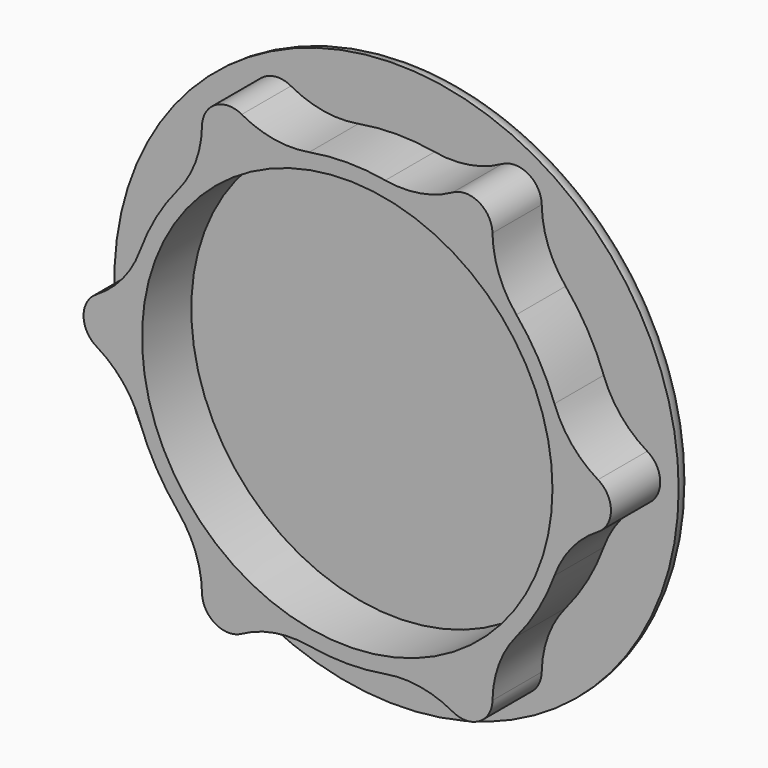
from build123d import *

# Parameters (mm, degrees)
F0_R     = 10
F1_DEPTH = 3
F2_R     = 13.75
F3_DEPTH = 1
F4_R     = 0.99999


# Not quite as in the source:
# - a fillet or chamfer is up to 0.001 mm smaller than in the source, because OpenCascade refuses the exact size


with BuildPart() as f1:
    # F0 (on Front) → F1 (new body)
    with BuildSketch(Plane.XZ):
        with BuildLine():
            ThreePointArc((-7.0762930266, 10.0230719262), (-7.391479251, 8.3623594503), (-8.2420141709, 6.901572459))
            ThreePointArc((-8.2420141709, 6.901572459), (-9.3097730907, 5.375), (-10.097944161, 3.6870074208))
            ThreePointArc((-10.097944161, 3.6870074208), (-10.937755345, 2.2200290777), (-12.2183814254, 1.1167135625))
            ThreePointArc((-12.2183814254, 1.1167135625), (-12.85, 0), (-12.2183814254, -1.1167135625))
            ThreePointArc((-12.2183814254, -1.1167135625), (-10.937755345, -2.2200290777), (-10.097944161, -3.6870074208))
            ThreePointArc((-10.097944161, -3.6870074208), (-9.3097730907, -5.375), (-8.2420141709, -6.901572459))
            ThreePointArc((-8.2420141709, -6.901572459), (-7.391479251, -8.3623594503), (-7.0762930266, -10.0230719262))
            ThreePointArc((-7.0762930266, -10.0230719262), (-6.425, -11.1284264386), (-5.1420883988, -11.1397854887))
            ThreePointArc((-5.1420883988, -11.1397854887), (-3.5462760941, -10.582388528), (-1.8559299902, -10.5885798798))
            ThreePointArc((-1.8559299902, -10.5885798798), (0, -10.75), (1.8559299902, -10.5885798798))
            ThreePointArc((1.8559299902, -10.5885798798), (3.5462760941, -10.582388528), (5.1420883988, -11.1397854887))
            ThreePointArc((5.1420883988, -11.1397854887), (6.425, -11.1284264386), (7.0762930266, -10.0230719262))
            ThreePointArc((7.0762930266, -10.0230719262), (7.391479251, -8.3623594503), (8.2420141709, -6.901572459))
            ThreePointArc((8.2420141709, -6.901572459), (9.3097730907, -5.375), (10.097944161, -3.6870074208))
            ThreePointArc((10.097944161, -3.6870074208), (10.937755345, -2.2200290777), (12.2183814254, -1.1167135625))
            ThreePointArc((12.2183814254, -1.1167135625), (12.85, 0), (12.2183814254, 1.1167135625))
            ThreePointArc((12.2183814254, 1.1167135625), (10.937755345, 2.2200290777), (10.097944161, 3.6870074208))
            ThreePointArc((10.097944161, 3.6870074208), (9.3097730907, 5.375), (8.2420141709, 6.901572459))
            ThreePointArc((8.2420141709, 6.901572459), (7.391479251, 8.3623594503), (7.0762930266, 10.0230719262))
            ThreePointArc((7.0762930266, 10.0230719262), (6.425, 11.1284264386), (5.1420883988, 11.1397854887))
            ThreePointArc((5.1420883988, 11.1397854887), (3.5462760941, 10.582388528), (1.8559299902, 10.5885798798))
            ThreePointArc((1.8559299902, 10.5885798798), (0, 10.75), (-1.8559299902, 10.5885798798))
            ThreePointArc((-1.8559299902, 10.5885798798), (-3.5462760941, 10.582388528), (-5.1420883988, 11.1397854887))
            ThreePointArc((-5.1420883988, 11.1397854887), (-6.425, 11.1284264386), (-7.0762930266, 10.0230719262))
        make_face()
        Circle(F0_R, mode=Mode.SUBTRACT)
    extrude(amount=F1_DEPTH)

    # F2 (on Front) → F3 (join)
    with BuildSketch(Plane.XZ):
        Circle(F2_R)
    extrude(amount=-F3_DEPTH)

    # F4 (radius 1 in the source; OpenCascade refuses exactly that, so slightly less here)
    f4_edges = [f1.edges().sort_by_distance(p)[0] for p in [
        (-13.75, 1, 0),
    ]]
    fillet(f4_edges, radius=F4_R)


solid = f1.part
